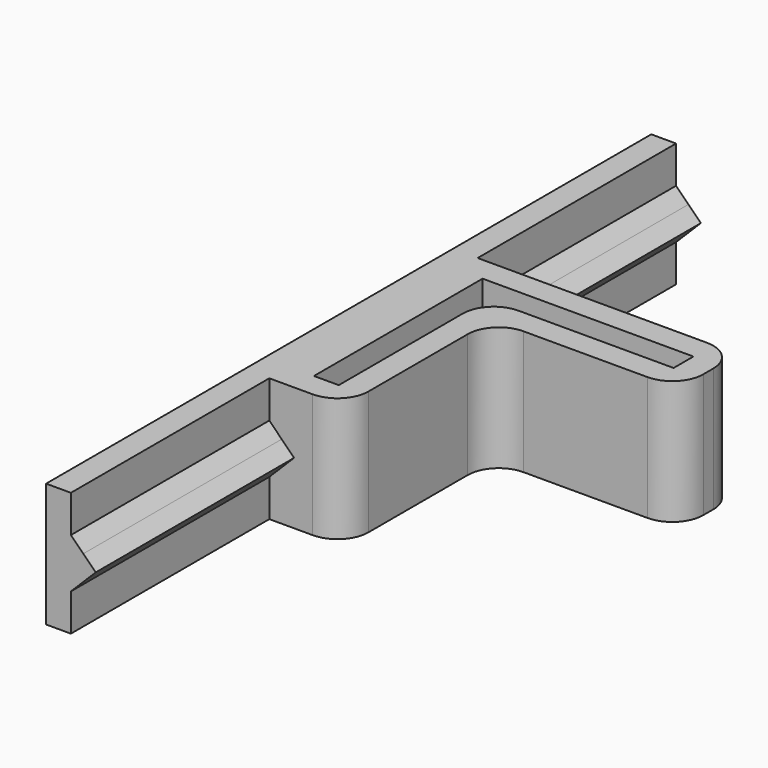
from build123d import *

# Parameters (mm, degrees)
F1_DEPTH = 12.7
F2_R     = 3.175
F3_W     = 77.47
F3_H     = 12.7
F4_DEPTH = 2.54
F5_W     = 25.4
F5_H     = 2.54
F6_DEPTH = 2.54
F7_SIZE  = 1.26999


# Not quite as in the source:
# - a fillet or chamfer is up to 0.001 mm smaller than in the source, because OpenCascade refuses the exact size


with BuildPart() as f1:
    # F0 (on Top) → F1 (new body)
    with BuildSketch(Plane.XY):
        Polygon((0, 24.13), (0, -2.1948770154), (0, -2.54), (7.62, -2.54), (7.62, 16.51), (26.67, 16.51), (26.67, 24.13), align=None)
        Polygon((5.08, 0), (2.54, 0), (2.54, 21.59), (5.08, 21.59), (24.13, 21.59), (24.13, 19.05), (5.08, 19.05), align=None, mode=Mode.SUBTRACT)
    extrude(amount=F1_DEPTH)

    # F2
    f2_edges = [f1.edges().sort_by_distance(p)[0] for p in [
        (26.67, 24.13, 6.35),
        (26.67, 16.51, 6.35),
        (5.08, 19.05, 6.35),
        (7.62, -2.54, 6.35),
        (7.62, 16.51, 6.35),
    ]]
    fillet(f2_edges, radius=F2_R)

    # F3 (on face) → F4 (join)
    with BuildSketch(Plane(origin=(0, 0, 0), x_dir=(0, -1, 0), z_dir=(-1, 0, 0))):
        with Locations((-10.795, 6.35)):
            Rectangle(F3_W, F3_H)
    extrude(amount=F4_DEPTH)

    # F5 (on face) → F6 (join)
    with BuildSketch(Plane.YZ):
        with Locations((36.83, 6.35)):
            Rectangle(F5_W, F5_H)
        with Locations((-15.24, 6.35)):
            Rectangle(F5_W, F5_H)
    extrude(amount=F6_DEPTH)

    # F7 (size 1.27 in the source; OpenCascade refuses exactly that, so slightly less here)
    f7_edges = [f1.edges().sort_by_distance(p)[0] for p in [
        (2.54, -15.24, 5.08),
        (2.54, -15.24, 7.62),
        (2.54, 36.83, 7.62),
        (2.54, 36.83, 5.08),
        (0, -15.24, 5.08),
        (0, -15.24, 7.62),
        (0, 36.83, 7.62),
        (0, 36.83, 5.08),
    ]]
    chamfer(f7_edges, length=F7_SIZE)


solid = f1.part
